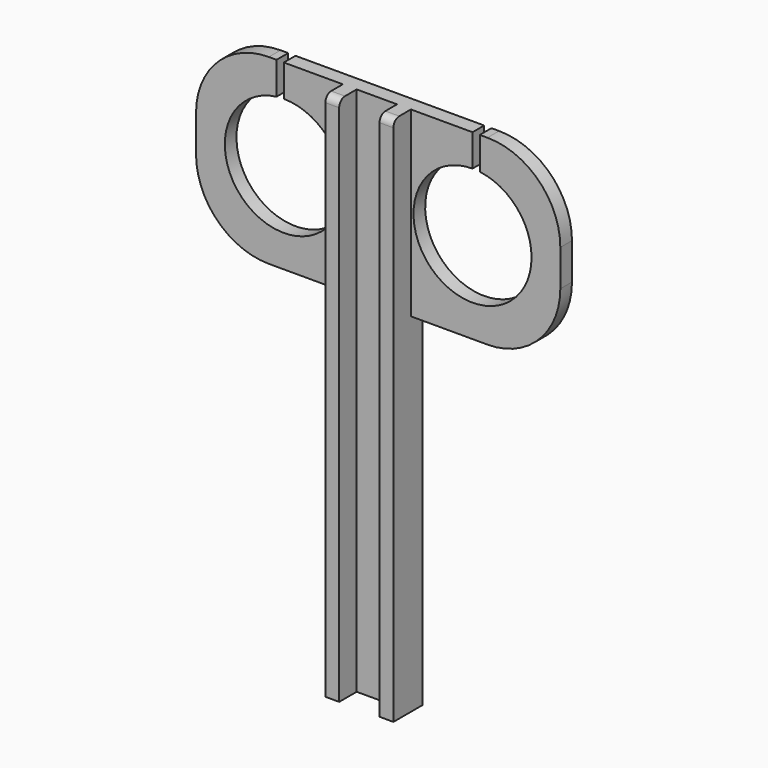
from build123d import *

# Parameters (mm, degrees)
F0_W     = 5.54
F0_H     = 25
F1_DEPTH = 2
F2_R     = 10
F3_DEPTH = 5
F5_DEPTH = 47.79
F6_R     = 1


# Not quite as in the source:
# - a feature of the source that left no trace in its solid (it failed there, or was rolled back) is left out


with BuildPart() as f1:
    # F0 (on Front) → F1 (new body)
    with BuildSketch(Plane.XZ):
        with BuildLine():
            Line((4.49, -12.5), (25, -12.5))
            Line((25, -12.5), (25, 12.5))
            Line((25, 12.5), (13.95, 12.5))
            Line((13.95, 12.5), (13.95, 8.0380345856))
            ThreePointArc((13.95, 8.0380345856), (19.0208319035, 5.3623688795), (21.05, 0))
            ThreePointArc((21.05, 0), (7.2224350724, -5.7275649276), (12.95, 8.1))
            Line((12.95, 8.1), (12.95, 12.5))
            Line((12.95, 12.5), (4.49, 12.5))
            Line((4.49, 12.5), (4.49, 0))
            Line((4.49, 0), (4.49, -12.5))
        make_face()
        with BuildLine():
            ThreePointArc((-12.95, 8.1), (-7.2224350724, 5.7275649276), (-4.85, 0))
            Line((-4.85, 0), (-4.85, 12.5))
            Line((-4.85, 12.5), (-12.95, 12.5))
            Line((-12.95, 12.5), (-12.95, 8.1))
        make_face()
        with BuildLine():
            Line((-25, -12.5), (-4.85, -12.5))
            Line((-4.85, -12.5), (-4.85, 0))
            ThreePointArc((-4.85, 0), (-18.3123688795, -6.0708319035), (-13.95, 8.0380345856))
            Line((-13.95, 8.0380345856), (-13.95, 12.5))
            Line((-13.95, 12.5), (-25, 12.5))
            Line((-25, 12.5), (-25, -12.5))
        make_face()
        Polygon((-4.85, -12.5), (-2.95, -12.5), (-2.95, 12.5), (-4.85, 12.5), (-4.85, 0), align=None)
        with Locations((-0.18, 0)):
            Rectangle(F0_W, F0_H)
        Polygon((2.59, -12.5), (4.49, -12.5), (4.49, 0), (4.49, 12.5), (2.59, 12.5), align=None)
    extrude(amount=F1_DEPTH)

    # F2
    f2_edges = [f1.edges().sort_by_distance(p)[0] for p in [
        (25, -1, -12.5),
        (25, -1, 12.5),
        (-25, -1, 12.5),
        (-25, -1, -12.5),
    ]]
    fillet(f2_edges, radius=F2_R)

    # F0 (on Front) → F3 (join)
    with BuildSketch(Plane.XZ):
        Polygon((2.59, -12.5), (4.49, -12.5), (4.49, 0), (4.49, 12.5), (2.59, 12.5), align=None)
        Polygon((-4.85, -12.5), (-2.95, -12.5), (-2.95, 12.5), (-4.85, 12.5), (-4.85, 0), align=None)
    extrude(amount=F3_DEPTH)

    # F4 (on face) → F5 (join)
    with BuildSketch(Plane(origin=(0, 0, -12.5), x_dir=(1, 0, 0), z_dir=(0, 0, -1))):
        Polygon((-2.95, 5), (-4.85, 5), (-4.85, 0), (4.49, 0), (4.49, 2), (4.49, 5), (2.59, 5), (2.59, 2), (-2.95, 2), align=None)
    extrude(amount=F5_DEPTH)

    # F6
    f6_edges = [f1.edges().sort_by_distance(p)[0] for p in [
        (-3.9, -5, 12.5),
        (3.54, -5, 12.5),
    ]]
    fillet(f6_edges, radius=F6_R)


solid = f1.part
